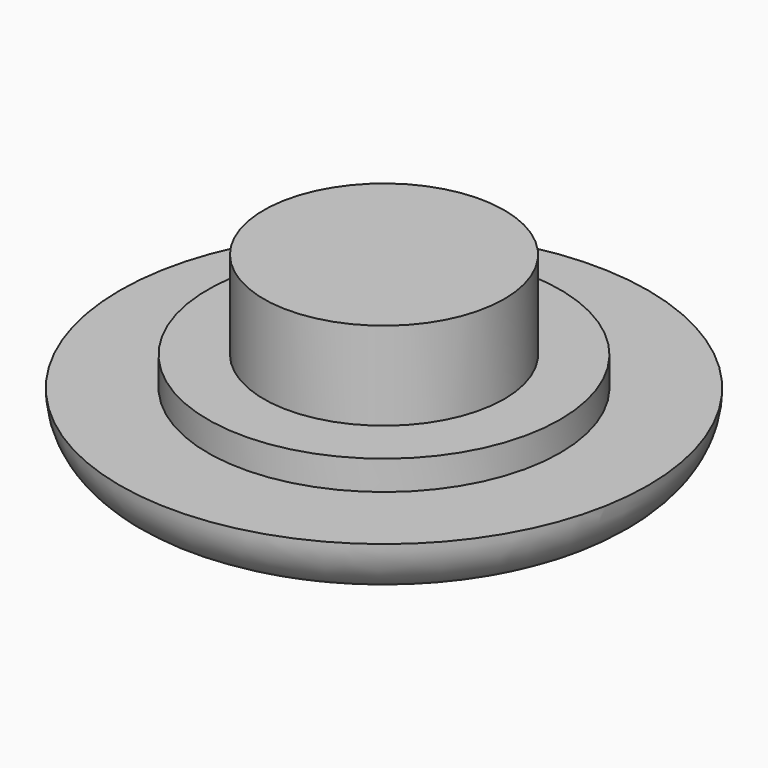
from build123d import *

# Parameters (mm, degrees)
F0_R     = 4.5
F1_DEPTH = 1
F2_R     = 3
F3_DEPTH = 0.5
F4_R     = 2.05
F5_DEPTH = 1.5
F6_R     = 0.99999


# Not quite as in the source:
# - a fillet or chamfer is up to 0.001 mm smaller than in the source, because OpenCascade refuses the exact size


with BuildPart() as f1:
    # F0 (on Top) → F1 (new body)
    with BuildSketch(Plane.XY):
        Circle(F0_R)
    extrude(amount=F1_DEPTH)

    # F2 (on face) → F3 (join)
    with BuildSketch(Plane.XY.offset(1)):
        Circle(F2_R)
    extrude(amount=F3_DEPTH)

    # F4 (on face) → F5 (join)
    with BuildSketch(Plane.XY.offset(1.5)):
        Circle(F4_R)
    extrude(amount=F5_DEPTH)

    # F6 (radius 1 in the source; OpenCascade refuses exactly that, so slightly less here)
    f6_edges = [f1.edges().sort_by_distance(p)[0] for p in [
        (-4.5, 0, 0),
    ]]
    fillet(f6_edges, radius=F6_R)


solid = f1.part
